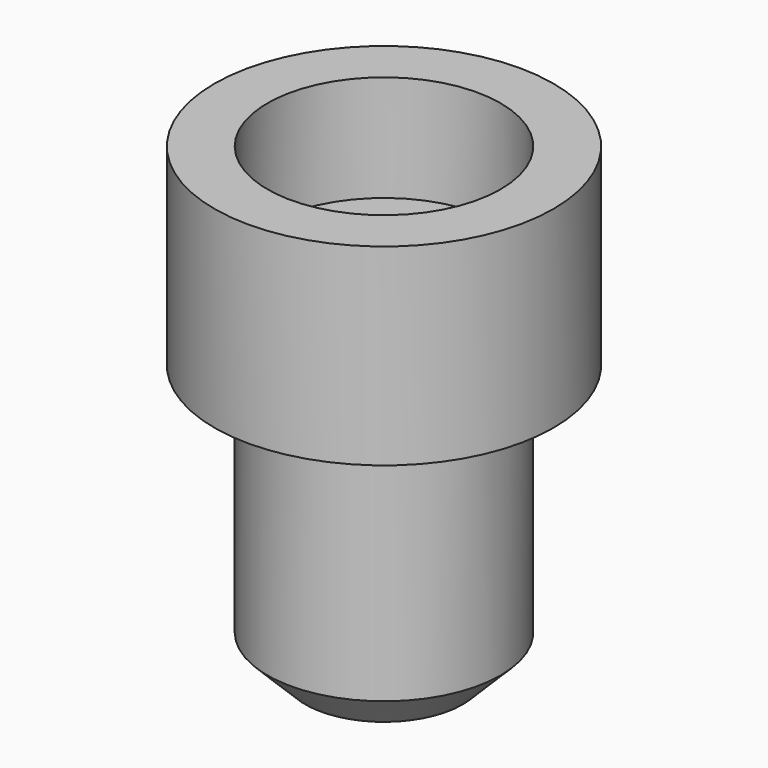
from build123d import *

# Parameters (mm, degrees)
F0_R     = 11.175
F0_R_2   = 7.6835
F1_DEPTH = 12.7
F2_DEPTH = 18
F3_DEPTH = 5.7
F4_SIZE  = 2.5


# Not quite as in the source:
# - a length typed as a fraction of an inch, garbled in the dataset ("3 / 203.2 mm" for 3/8 in), is restored


with BuildPart() as f1:
    # F0 (on Top) → F1 (new body)
    with BuildSketch(Plane.XY):
        Circle(F0_R)
        Circle(F0_R_2, mode=Mode.SUBTRACT)
    extrude(amount=F1_DEPTH)



with BuildPart() as f2:
    # F0 (on Top) → F2 (new body)
    with BuildSketch(Plane.XY):
        Circle(F0_R_2)
    extrude(amount=-F2_DEPTH)


with BuildPart() as f1_1:
    add(f1.part)

    add(f2.part)  # F3 merges F2
    # F0 (on Top) → F3 (join)
    with BuildSketch(Plane.XY):
        Circle(F0_R_2)
    extrude(amount=F3_DEPTH)

    # F4
    f4_edges = [f1_1.edges().sort_by_distance(p)[0] for p in [
        (-7.6835, 0, -18),
    ]]
    chamfer(f4_edges, length=F4_SIZE)


solid = f1_1.part
